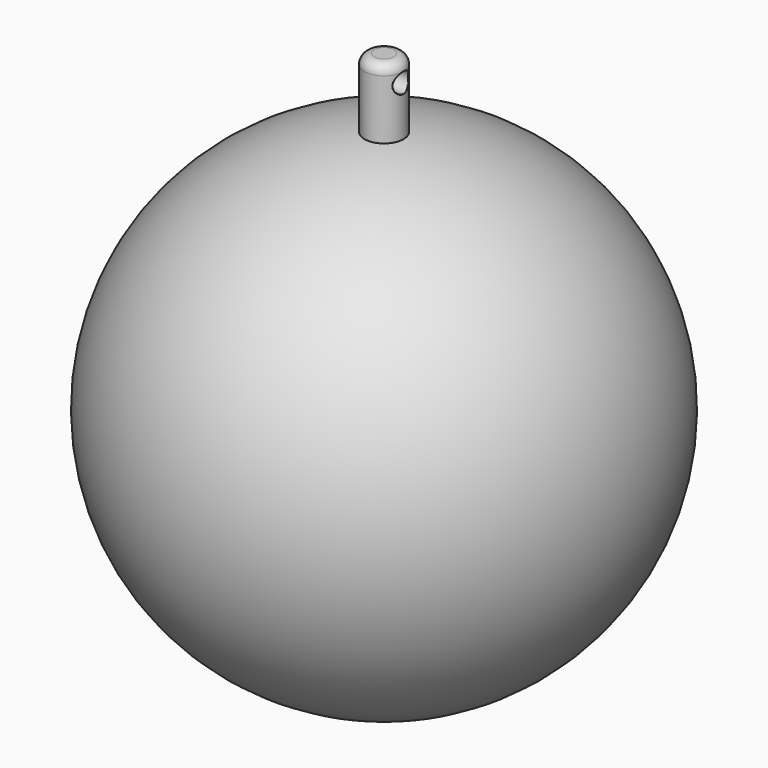
from build123d import *

# Parameters (mm, degrees)
F4_R     = 2
F5_DEPTH = 12.5
F6_R     = 1.99999
F7_R     = 0.1


# Not quite as in the source:
# - a fillet or chamfer is up to 0.001 mm smaller than in the source, because OpenCascade refuses the exact size


with BuildPart() as f1:
    # F0 (on Front) → F1 (revolve)
    with BuildSketch(Plane.XZ):
        with BuildLine():
            Line((0, 49.5), (0, 50))
            ThreePointArc((0, 50), (-50, 0), (0, -50))
            Line((0, -50), (0, -49.5))
            ThreePointArc((0, -49.5), (-49.5, 0), (0, 49.5))
        make_face()
    revolve(axis=Axis((0, 0, 0), (0, 0, -1)))


with BuildPart() as f3:
    # F2 (on Right) → F3 (revolve)
    with BuildSketch(Plane.YZ):
        with BuildLine():
            ThreePointArc((-4, 49.8397431775), (-2.001604497, 49.9599197301), (0, 50))
            Line((0, 50), (0, 64))
            Line((0, 64), (-4, 64))
            Line((-4, 64), (-4, 49.8397431775))
        make_face()
    revolve(axis=Axis((0, 0, 56.9119527936), (0, 0, 1)))

    # F4 (on Right) → F5 (cut, symmetric)
    with BuildSketch(Plane.YZ):
        with Locations((0, 60)):
            Circle(F4_R)
    extrude(amount=F5_DEPTH, both=True, mode=Mode.SUBTRACT)

    # F6 (radius 2 in the source; OpenCascade refuses exactly that, so slightly less here)
    f6_edges = [f3.edges().sort_by_distance(p)[0] for p in [
        (0, 4, 64),
    ]]
    fillet(f6_edges, radius=F6_R)

    # F7
    f7_edges = [f3.edges().sort_by_distance(p)[0] for p in [
        (3.464102, -2, 60),
    ]]
    fillet(f7_edges, radius=F7_R)


solid = Compound([f1.part, f3.part])
